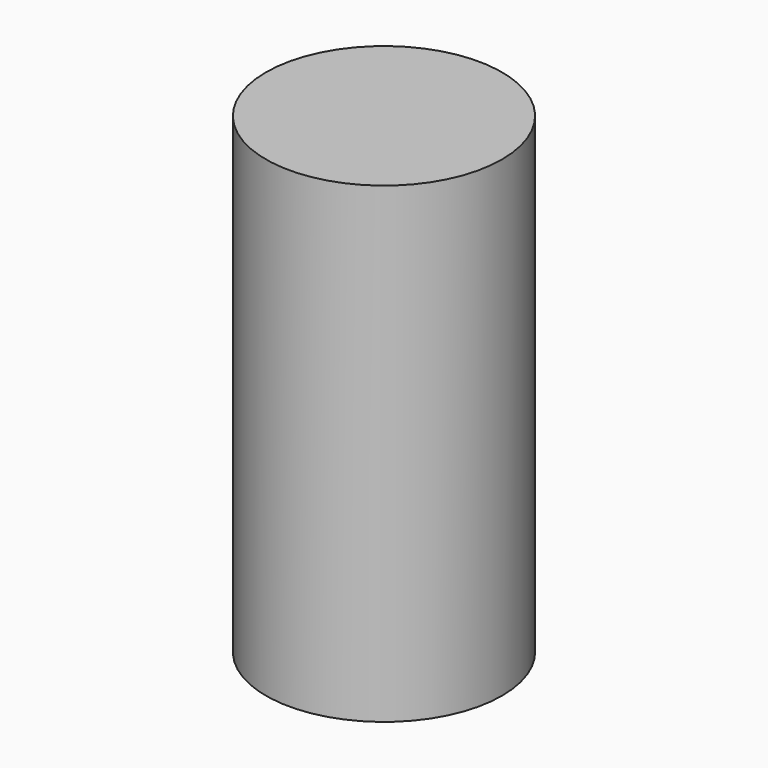
from build123d import *

# Parameters (mm, degrees)
F0_R        = 5.5
F0_R_2      = 5
F1_DEPTH    = 20
F2_DEPTH    = 2
F3_R        = 0.5
F4_T1_DEPTH = 3.6258666345
F4_T3_DEPTH = 3.25
F4_T5_DEPTH = 2.959158735


# Not quite as in the source:
# - a fillet or chamfer that OpenCascade refuses, or shapes differently, is made with other operations: its cross-section is extruded or revolved along the edge and cut away or added
# - a feature names something its author has since deleted; it is built from what else it names


with BuildPart() as f1:
    # F0 (on Top) → F1 (new body)
    with BuildSketch(Plane.XY):
        with Locations((1.0606649963, 0)):
            Circle(F0_R)
        with Locations((1.0606649963, 0)):
            Circle(F0_R_2, mode=Mode.SUBTRACT)
        with Locations((1.0606649963, 0)):
            Circle(F0_R_2)
        Polygon((-1.4393350037, -3.5), (-2.4393350037, -3.5), (-2.4393350037, 2.6), (0.6516276405, 3.4282209443), (0.6516276405, 2.4282209443), (-1.4393350037, 1.8679491924), (-1.4393350037, 0.8042534147), (0.0095537358, 1.1924819824), (0.0095537358, 0.1924819824), (-1.4393350037, -0.1957465853), align=None, mode=Mode.SUBTRACT)
        Polygon((1.5606649963, -3.5), (1.5606649963, 2.6), (4.6516276405, 3.4282209443), (4.6516276405, 2.4282209443), (2.5606649963, 1.8679491924), (2.5606649963, 0.8042534147), (4.0095537358, 1.1924819824), (4.0095537358, 0.1924819824), (2.5606649963, -0.1957465853), (2.5606649963, -3.5), align=None, mode=Mode.SUBTRACT)
        Polygon((4.6516276405, 3.4282209443), (1.5606649963, 2.6), (1.5606649963, -3.5), (2.5606649963, -3.5), (2.5606649963, -0.1957465853), (4.0095537358, 0.1924819824), (4.0095537358, 1.1924819824), (2.5606649963, 0.8042534147), (2.5606649963, 1.8679491924), (4.6516276405, 2.4282209443), align=None)
        Polygon((-2.4393350037, 2.6), (-2.4393350037, -3.5), (-1.4393350037, -3.5), (-1.4393350037, -0.1957465853), (0.0095537358, 0.1924819824), (0.0095537358, 1.1924819824), (-1.4393350037, 0.8042534147), (-1.4393350037, 1.8679491924), (0.6516276405, 2.4282209443), (0.6516276405, 3.4282209443), align=None)
    extrude(amount=F1_DEPTH)

    # F0 (on Top) → F2 (join)
    with BuildSketch(Plane.XY):
        with Locations((1.0606649963, 0)):
            Circle(F0_R)
        with Locations((1.0606649963, 0)):
            Circle(F0_R_2, mode=Mode.SUBTRACT)
        Polygon((-2.4393350037, 2.6), (-2.4393350037, -3.5), (-1.4393350037, -3.5), (-1.4393350037, -0.1957465853), (0.0095537358, 0.1924819824), (0.0095537358, 1.1924819824), (-1.4393350037, 0.8042534147), (-1.4393350037, 1.8679491924), (0.6516276405, 2.4282209443), (0.6516276405, 3.4282209443), align=None)
        Polygon((4.6516276405, 3.4282209443), (1.5606649963, 2.6), (1.5606649963, -3.5), (2.5606649963, -3.5), (2.5606649963, -0.1957465853), (4.0095537358, 0.1924819824), (4.0095537358, 1.1924819824), (2.5606649963, 0.8042534147), (2.5606649963, 1.8679491924), (4.6516276405, 2.4282209443), align=None)
    extrude(amount=-F2_DEPTH)

    # F3
    f3_edges = [f1.edges().sort_by_distance(p)[0] for p in [
        (2.560665, -3.5, -1),
        (-1.439335, -3.5, -1),
        (4.009554, 0.192482, -1),
        (0.009554, 0.192482, -1),
        (4.651628, 2.428221, -1),
        (0.651628, 2.428221, -1),
    ]]
    fillet(f3_edges, radius=F3_R)

    # F4: fillet of radius 0.5 on 8 edges, made by hand

    # F4_s2 → F4_t1 (cut)
    with BuildSketch(Plane.XY.offset(-3.6258666345)):
        with BuildLine():
            ThreePointArc((4.6516276405, 2.8118844383), (4.4431733372, 3.1840141424), (4.0234410115, 3.2598988444))
            Line((4.0234410115, 3.2598988444), (4.6516276405, 3.4282209443))
            Line((4.6516276405, 3.4282209443), (4.6516276405, 2.8118844383))
        make_face()
        with BuildLine():
            ThreePointArc((0.0234410115, 3.2598988444), (0.4431733372, 3.1840141424), (0.6516276405, 2.8118844383))
            Line((0.6516276405, 2.8118844383), (0.6516276405, 3.4282209443))
            Line((0.6516276405, 3.4282209443), (0.0234410115, 3.2598988444))
        make_face()
        with BuildLine():
            ThreePointArc((0.0095537358, 0.5761454764), (-0.1989005675, 0.9482751804), (-0.6186328932, 1.0241598824))
            Line((-0.6186328932, 1.0241598824), (0.0095537358, 1.1924819824))
            Line((0.0095537358, 1.1924819824), (0.0095537358, 0.5761454764))
        make_face()
        with BuildLine():
            ThreePointArc((3.3813671068, 1.0241598824), (3.8010994325, 0.9482751804), (4.0095537358, 0.5761454764))
            Line((4.0095537358, 0.5761454764), (4.0095537358, 1.1924819824))
            Line((4.0095537358, 1.1924819824), (3.3813671068, 1.0241598824))
        make_face()
    extrude(amount=F4_T1_DEPTH, mode=Mode.SUBTRACT)

    # F4_s4 → F4_t3 (cut)
    with BuildSketch(Plane.XY.offset(-3.25)):
        with BuildLine():
            ThreePointArc((1.5606649963, -3), (1.7071116058, -3.3535533906), (2.0606649963, -3.5))
            Line((2.0606649963, -3.5), (1.5606649963, -3.5))
            Line((1.5606649963, -3.5), (1.5606649963, -3))
        make_face()
        with BuildLine():
            ThreePointArc((-1.9393350037, -3.5), (-2.2928883942, -3.3535533906), (-2.4393350037, -3))
            Line((-2.4393350037, -3), (-2.4393350037, -3.5))
            Line((-2.4393350037, -3.5), (-1.9393350037, -3.5))
        make_face()
    extrude(amount=F4_T3_DEPTH, mode=Mode.SUBTRACT)

    # F4_s6 → F4_t5 (cut)
    with BuildSketch(Plane.XY.offset(-2.959158735)):
        with BuildLine():
            ThreePointArc((1.9312554738, 2.6992994192), (1.6639883262, 2.5207172205), (1.5606649963, 2.216336506))
            Line((1.5606649963, 2.216336506), (1.5606649963, 2.6))
            Line((1.5606649963, 2.6), (1.9312554738, 2.6992994192))
        make_face()
        with BuildLine():
            ThreePointArc((-2.4393350037, 2.216336506), (-2.3360116738, 2.5207172205), (-2.0687445262, 2.6992994192))
            Line((-2.0687445262, 2.6992994192), (-2.4393350037, 2.6))
            Line((-2.4393350037, 2.6), (-2.4393350037, 2.216336506))
        make_face()
    extrude(amount=F4_T5_DEPTH, mode=Mode.SUBTRACT)


solid = f1.part
